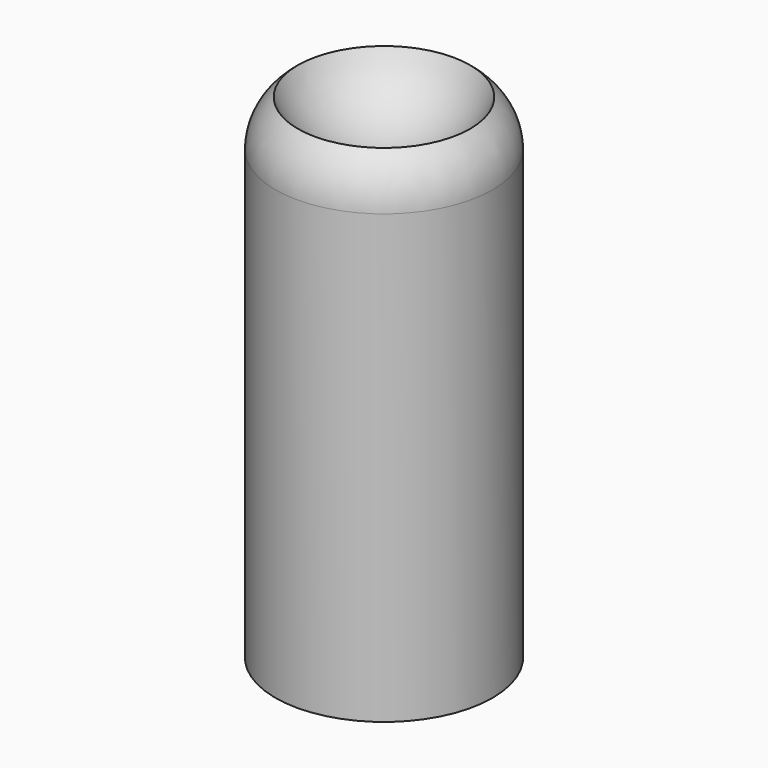
from build123d import *

# Parameters (mm, degrees)
F0_R     = 5.5
F0_R_2   = 3.85
F1_DEPTH = 25
F2_START = 11
F2_DEPTH = 14


# Not quite as in the source:
# - a fillet or chamfer that OpenCascade refuses, or shapes differently, is made with other operations: its cross-section is extruded or revolved along the edge and cut away or added


with BuildPart() as f1:
    # F0 (on Top) → F1 (new body)
    with BuildSketch(Plane.XY):
        Circle(F0_R)
        Circle(F0_R_2, mode=Mode.SUBTRACT)
    extrude(amount=F1_DEPTH)

    # F0 (on Top) → F2 (join)
    with BuildSketch(Plane.XY.offset(F2_START)):
        Circle(F0_R_2)
    extrude(amount=F2_DEPTH)

    # F3 (on Front) → F4 (revolve, cut)
    with BuildSketch(Plane.XZ):
        with BuildLine():
            Line((0, 22.2), (0, 31.8))
            ThreePointArc((0, 31.8), (-4.8, 27), (0, 22.2))
        make_face()
    revolve(axis=Axis((0, 0, 27), (0, 0, -1)), mode=Mode.SUBTRACT)

    # F5: fillet of radius 3 on 1 edges, made by hand

    # F5_s1 → F5_t2 (revolve, cut)
    with BuildSketch(Plane.XZ):
        with BuildLine():
            ThreePointArc((5.5, 22.6489525251), (5.2009678393, 23.9546219822), (4.3634848459, 25))
            Line((4.3634848459, 25), (5.5, 25))
            Line((5.5, 25), (5.5, 22.6489525251))
        make_face()
    revolve(axis=Axis((0, 0, 25), (0, 0, 1)), mode=Mode.SUBTRACT)


solid = f1.part
